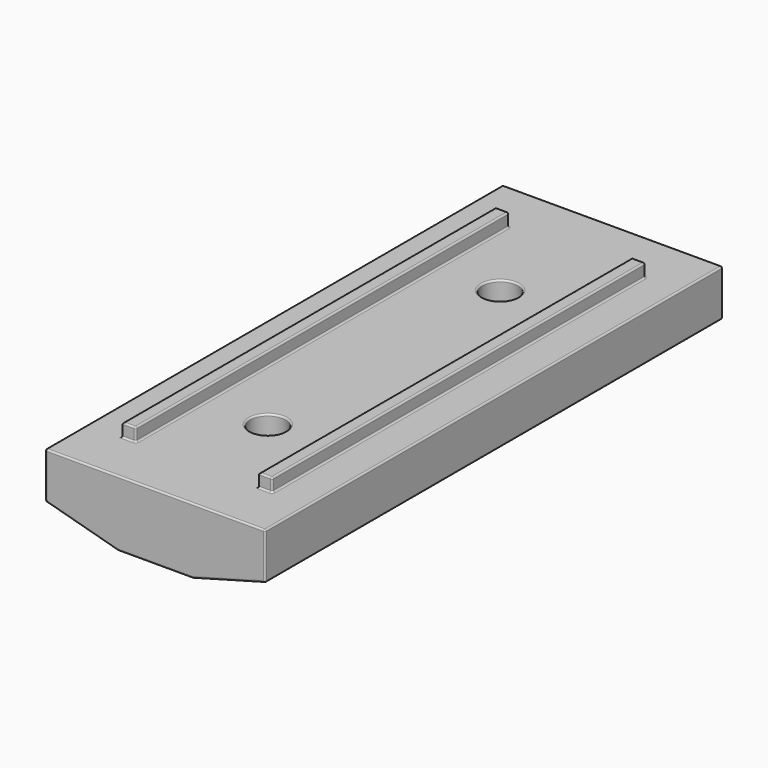
from build123d import *

# Parameters (mm, degrees)
F0_W     = 635
F0_H     = 1651
F1_DEPTH = 190.5
F3_DEPTH = 1651.001
F4_W     = 38.1
F4_H     = 1346.2
F5_DEPTH = 38.1
F7_R     = 50.8
F8_DEPTH = 190.501
F8_TAPER = -3
F9_R     = 4.7625


with BuildPart() as f1:
    # F0 (on Top) → F1 (new body)
    with BuildSketch(Plane.XY):
        Rectangle(F0_W, F0_H)
    extrude(amount=F1_DEPTH)

    # F2 (on face) → F3 (cut, through all)
    with BuildSketch(Plane.XZ.offset(825.5)):
        Polygon((317.5, 57.15), (107.95, 0), (317.5, 0), align=None)
        Polygon((-317.5, 0), (-107.95, 0), (-317.5, 57.15), align=None)
    extrude(amount=-F3_DEPTH, mode=Mode.SUBTRACT)

    # F4 (on face) → F5 (join)
    with BuildSketch(Plane.XY.offset(190.5)):
        with Locations((-196.85, 0)):
            Rectangle(F4_W, F4_H)
        with Locations((196.85, 0)):
            Rectangle(F4_W, F4_H)
    extrude(amount=F5_DEPTH)

    # F7 (on face) → F8 (cut, through all)
    with BuildSketch(Plane.XY.offset(190.5)):
        with Locations((0, -419.1)):
            Circle(F7_R)
        with Locations((0, 419.1)):
            Circle(F7_R)
    extrude(amount=-F8_DEPTH, taper=F8_TAPER, mode=Mode.SUBTRACT)

    # F9
    f9_edges = [f1.edges().sort_by_distance(p)[0] for p in [
        (-177.8, -673.1, 209.55),
        (-177.8, 673.1, 209.55),
        (-177.8, 0, 190.5),
        (-177.8, 0, 228.6),
        (-196.85, 673.1, 228.6),
        (-215.9, 0, 228.6),
        (-196.85, -673.1, 228.6),
        (215.9, -673.1, 209.55),
        (215.9, 673.1, 209.55),
        (215.9, 0, 190.5),
        (215.9, 0, 228.6),
        (196.85, 673.1, 228.6),
        (177.8, 0, 228.6),
        (196.85, -673.1, 228.6),
        (0, -825.5, 190.5),
        (-317.5, 0, 190.5),
        (317.5, 0, 190.5),
        (0, 825.5, 190.5),
        (-50.8, -419.1, 190.5),
        (-196.85, 673.1, 190.5),
        (-215.9, 0, 190.5),
        (-196.85, -673.1, 190.5),
        (196.85, 673.1, 190.5),
        (177.8, 0, 190.5),
        (196.85, -673.1, 190.5),
        (-50.8, 419.1, 190.5),
        (317.5, 0, 57.15),
        (317.5, 825.5, 123.825),
        (317.5, -825.5, 123.825),
        (-212.725, -825.5, 28.575),
        (0, -825.5, 0),
        (212.725, -825.5, 28.575),
        (-317.5, -825.5, 123.825),
        (212.725, 825.5, 28.575),
        (0, 825.5, 0),
        (-212.725, 825.5, 28.575),
        (-317.5, 825.5, 123.825),
        (-317.5, 0, 57.15),
        (-107.95, 0, 0),
        (107.95, 0, 0),
        (-60.783682, -419.1, 0),
        (-60.783682, 419.1, 0),
    ]]
    fillet(f9_edges, radius=F9_R)


solid = f1.part
